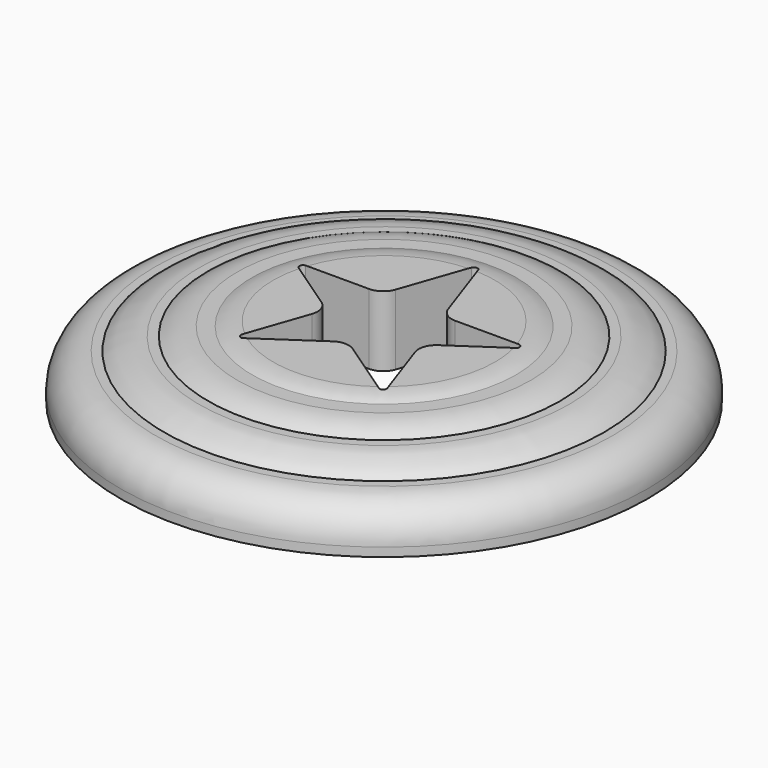
from build123d import *

# Parameters (mm, degrees)
F0_R      = 38.1
F1_DEPTH  = 3.175
F3_R      = 31.75
F4_DEPTH  = 1.905
F5_R      = 25.4
F6_DEPTH  = 1.27
F7_R      = 19.05
F8_DEPTH  = 0.635
F10_DEPTH = 10.161
F11_R     = 5.08
F15_R     = 2.54
F16_R     = 0.508


# Not quite as in the source:
# - a fillet or chamfer that OpenCascade refuses, or shapes differently, is made with other operations: its cross-section is extruded or revolved along the edge and cut away or added


with BuildPart() as f1:
    # F0 (on Top) → F1 (new body, symmetric)
    with BuildSketch(Plane.XY):
        Circle(F0_R)
    extrude(amount=F1_DEPTH, both=True)

    # F3 (on face) → F4 (join)
    with BuildSketch(Plane.XY.offset(3.175)):
        Circle(F3_R)
    extrude(amount=F4_DEPTH)

    # F5 (on face) → F6 (join)
    with BuildSketch(Plane.XY.offset(5.08)):
        Circle(F5_R)
    extrude(amount=F6_DEPTH)

    # F7 (on face) → F8 (join)
    with BuildSketch(Plane.XY.offset(6.35)):
        Circle(F7_R)
    extrude(amount=F8_DEPTH)

    # F9 (on face) → F10 (cut, through all)
    with BuildSketch(Plane(origin=(0, 0, -3.175), x_dir=(1, 0, 0), z_dir=(0, 0, -1))):
        Polygon((-6.8075360054, 1.8716637263), (-17.0388379885, -5.08), (-4.3994090512, -5.08), (0, -17.78), (4.3994090512, -5.08), (17.0388379885, -5.08), (6.8075360054, 1.8716637263), (10.9985226281, 13.97), (0, 6.4970477871), (-10.9985226281, 13.97), align=None)
    extrude(amount=-F10_DEPTH, mode=Mode.SUBTRACT)

    # F11
    f11_edges = [f1.edges().sort_by_distance(p)[0] for p in [
        (-38.1, 0, 3.175),
    ]]
    fillet(f11_edges, radius=F11_R)

    # F12: fillet of radius 7.62 on 1 edges, made by hand

    # F12_s1 → F12_t2 (revolve, cut)
    with BuildSketch(Plane.XZ):
        with BuildLine():
            ThreePointArc((31.75, 3.175), (29.4039205887, 4.5878573218), (26.7098437524, 5.08))
            Line((26.7098437524, 5.08), (31.75, 5.08))
            Line((31.75, 5.08), (31.75, 3.175))
        make_face()
    revolve(axis=Axis((0, 0, 5.08), (0, 0, 1)), mode=Mode.SUBTRACT)

    # F13: fillet of radius 7.62 on 1 edges, made by hand

    # F13_s1 → F13_t2 (revolve, cut)
    with BuildSketch(Plane.XZ):
        with BuildLine():
            ThreePointArc((25.4, 5.08), (23.3875910419, 6.0255945611), (21.1878865162, 6.35))
            Line((21.1878865162, 6.35), (25.4, 6.35))
            Line((25.4, 6.35), (25.4, 5.08))
        make_face()
    revolve(axis=Axis((0, 0, 6.35), (0, 0, 1)), mode=Mode.SUBTRACT)

    # F14: fillet of radius 7.62 on 1 edges, made by hand

    # F14_s1 → F14_t2 (revolve, cut)
    with BuildSketch(Plane.XZ):
        with BuildLine():
            ThreePointArc((16.0046469827, 6.985), (17.5600729694, 6.824560979), (19.05, 6.35))
            Line((19.05, 6.35), (19.05, 6.985))
            Line((19.05, 6.985), (16.0046469827, 6.985))
        make_face()
    revolve(axis=Axis((0, 0, 6.985), (0, 0, 1)), mode=Mode.SUBTRACT)

    # F15
    f15_edges = [f1.edges().sort_by_distance(p)[0] for p in [
        (4.399409, 5.08, 1.905),
        (-4.399409, 5.08, 1.905),
        (-6.807536, -1.871664, 1.905),
        (0, -6.497048, 1.905),
        (6.807536, -1.871664, 1.905),
    ]]
    fillet(f15_edges, radius=F15_R)

    # F16
    f16_edges = [f1.edges().sort_by_distance(p)[0] for p in [
        (-10.998523, -13.97, 1.800149),
        (-17.038838, 5.08, 1.800149),
        (0, 17.78, 1.800149),
        (17.038838, 5.08, 1.800149),
        (10.998523, -13.97, 1.800149),
    ]]
    fillet(f16_edges, radius=F16_R)


solid = f1.part
